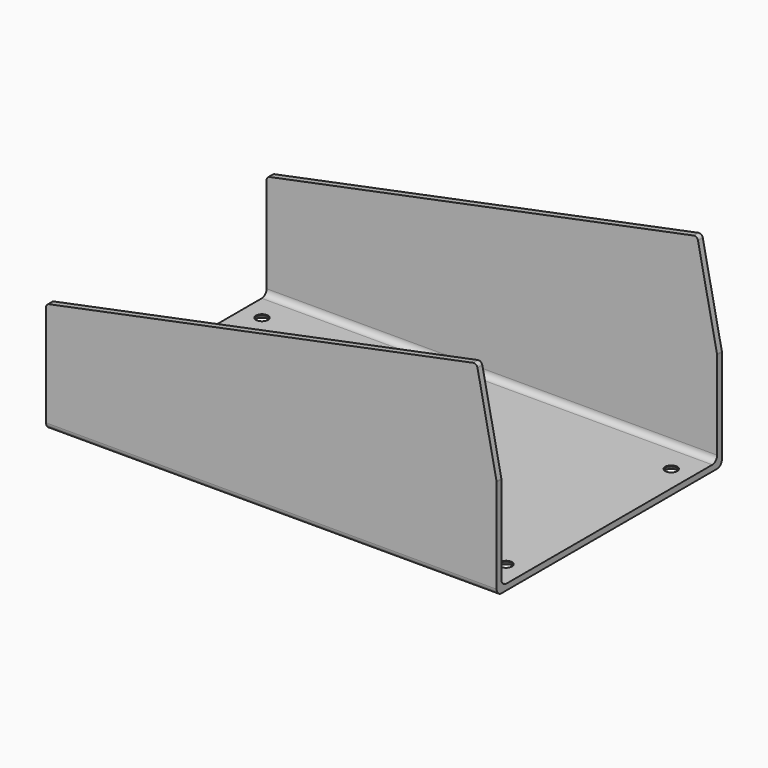
from build123d import *

# Parameters (mm, degrees)
F1_DEPTH       = 37.5
F2_T           = -1.6
F3_R           = 1.6
F5_D           = 3.2
F5_CSINK_D     = 6
F5_CSINK_ANGLE = 90
F6_R           = 1.6
F7_R           = 1


# Not quite as in the source:
# - a feature names something its author has since deleted; it is built from what else it names


with BuildPart() as f1:
    # F0 (on Front) → F1 (new body, symmetric)
    with BuildSketch(Plane.XZ):
        Polygon((-50.4974494928, -20.8124593111), (69.5025505072, -20.8124593111), (69.5025505072, 6.0025406889), (64.2012187523, 32.0403523478), (-50.4975286176, 8.6875406888), align=None)
    extrude(amount=F1_DEPTH, both=True)

    # F2
    f2_openings = [f1.faces().sort_by_distance(p)[0] for p in [
        (-50.497489, 0, -6.062459),
        (6.851845, 0, 20.363947),
        (66.851885, 0, 19.021447),
        (69.502551, 0, -7.404959),
    ]]
    offset(amount=F2_T, openings=f2_openings, kind=Kind.INTERSECTION)

    # F3
    f3_edges = [f1.edges().sort_by_distance(p)[0] for p in [
        (9.502548, -35.9, -19.212459),
        (9.502548, 35.9, -19.212459),
    ]]
    fillet(f3_edges, radius=F3_R)

    # F5 (through all)
    with Locations(Plane(origin=(0, 0, -20.8124593111), x_dir=(1, 0, 0), z_dir=(0, 0, -1))):
        with Locations((64.0025505072, -27.5), (-44.9974494928, -27.5), (64.0025505072, 27.5), (-44.9974494928, 27.5)):
            CounterSinkHole(F5_D / 2, F5_CSINK_D / 2, counter_sink_angle=F5_CSINK_ANGLE)

    # F6
    f6_edges = [f1.edges().sort_by_distance(p)[0] for p in [
        (9.502551, 37.5, -20.812459),
        (9.502551, -37.5, -20.812459),
    ]]
    fillet(f6_edges, radius=F6_R)

    # F7
    f7_edges = [f1.edges().sort_by_distance(p)[0] for p in [
        (64.201219, -36.7, 32.040352),
        (64.201219, 36.7, 32.040352),
        (69.502551, 36.7, 6.002541),
        (69.502551, -36.7, 6.002541),
        (-50.497529, -36.7, 8.687541),
        (-50.497529, 36.7, 8.687541),
    ]]
    fillet(f7_edges, radius=F7_R)


solid = f1.part
